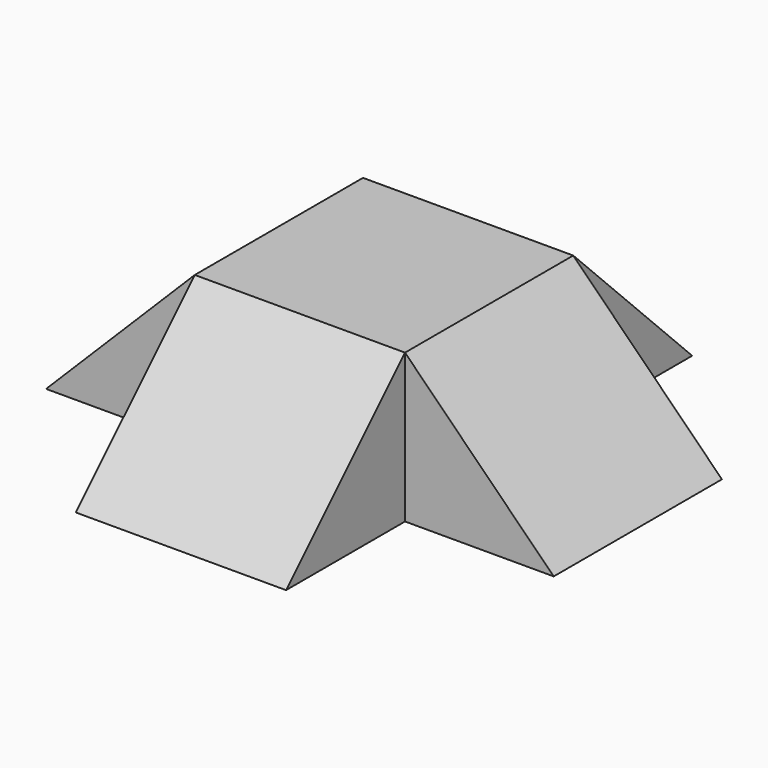
from build123d import *

# Parameters (mm, degrees)
F0_W     = 77.254
F0_H     = 22.627
F1_DEPTH = 16
F2_SIZE  = 22.62699
F4_COUNT = 2
F4_ANGLE = 90


# Not quite as in the source:
# - a fillet or chamfer is up to 0.001 mm smaller than in the source, because OpenCascade refuses the exact size


with BuildPart() as f1:
    # F0 (on Front) → F1 (new body, symmetric)
    with BuildSketch(Plane.XZ):
        Rectangle(F0_W, F0_H)
    extrude(amount=F1_DEPTH, both=True)

    # F2 (size 22.627 in the source; OpenCascade refuses exactly that, so slightly less here)
    f2_edges = [f1.edges().sort_by_distance(p)[0] for p in [
        (-38.627, 0, 11.3135),
        (38.627, 0, 11.3135),
    ]]
    chamfer(f2_edges, length=F2_SIZE)


with BuildPart() as f4_1:
    # F4: instance of F1
    add(f1.part.rotate(Axis((0, 0, -2.2350996733), (0, 0, 1)), 1 * F4_ANGLE / (F4_COUNT - 1)))


solid = Compound([f1.part, f4_1.part])
